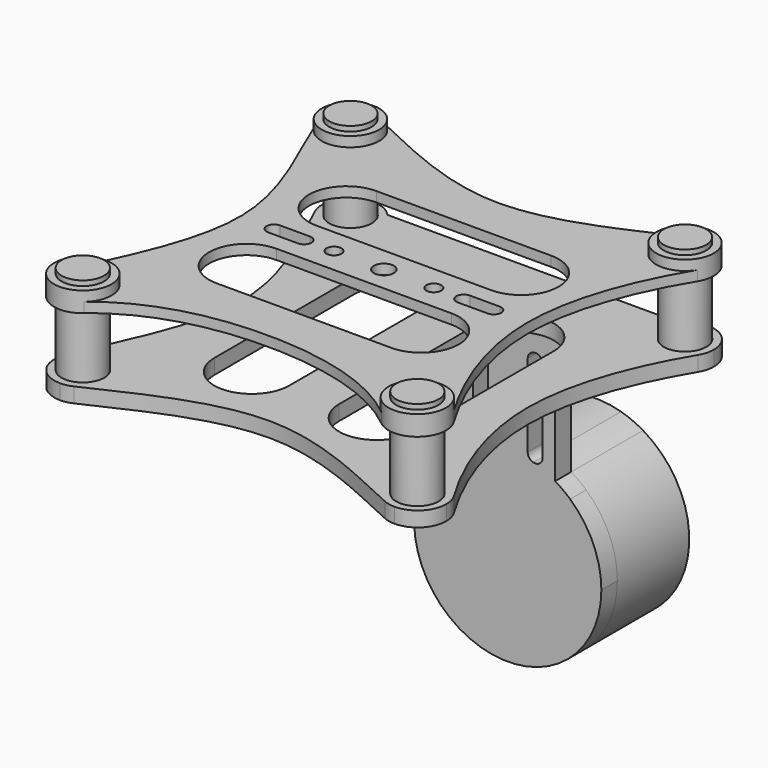
from build123d import *
from build123d import SkipClean  # not in build123d's __all__

# Parameters (mm, degrees)
F0_R          = 4.25
F0_R_2        = 1.5
F0_R_3        = 2
F1_DEPTH      = 2
F2_DEPTH      = 16
F2_DEPTH_BACK = 1
F3_R          = 4.25
F4_DEPTH      = 3
F6_START      = -31
F6_DEPTH      = 4
F8_DEPTH      = 18
F2_FACE1_R    = 4.25
F9_DEPTH      = 4


# Not quite as in the source:
# - after a boolean that leaves OpenCascade's solid faulty, fix() repairs it


with BuildPart() as f1:
    # F0 (on Top) → F1 (new body)
    with BuildSketch(Plane.XY):
        with BuildLine():
            ThreePointArc((33.5, -39.25), (37.5658639918, -37.5658639918), (39.25, -33.5))
            ThreePointArc((39.25, -33.5), (39.0420799623, -31.9677305421), (38.433356629, -30.5462748316))
            ThreePointArc((38.433356629, -30.5462748316), (29.7463089973, -29.1442791807), (29.8501801445, -37.9431199649))
            ThreePointArc((29.8501801445, -37.9431199649), (31.5616295243, -38.9134295875), (33.5, -39.25))
        make_face()
        with Locations((33.5, -33.5)):
            Circle(F0_R, mode=Mode.SUBTRACT)
        with BuildLine():
            ThreePointArc((-38.7378752338, -31.1278357908), (-39.1205107683, -32.2865921119), (-39.25, -33.5))
            ThreePointArc((-39.25, -33.5), (-37.5658639918, -37.5658639918), (-33.5, -39.25))
            ThreePointArc((-33.5, -39.25), (-31.5124151451, -38.8955543223), (-29.7698705896, -37.875915285))
            ThreePointArc((-29.7698705896, -37.875915285), (-28.2793322214, -35.9097983204), (-27.75, -33.5))
            ThreePointArc((-27.75, -33.5), (-32.2865921119, -27.8794892317), (-38.7378752338, -31.1278357908))
        make_face()
        with Locations((-33.5, -33.5)):
            Circle(F0_R, mode=Mode.SUBTRACT)
        with BuildLine():
            ThreePointArc((-31.0866116343, 38.7190091585), (-32.2644439837, 39.1156835141), (-33.5, 39.25))
            ThreePointArc((-33.5, 39.25), (-37.5658639918, 37.5658639918), (-39.25, 33.5))
            ThreePointArc((-39.25, 33.5), (-39.1467228333, 32.4150939007), (-38.8406013064, 31.369160333))
            ThreePointArc((-38.8406013064, 31.369160333), (-32.4150939007, 27.8532771667), (-27.75, 33.5))
            ThreePointArc((-27.75, 33.5), (-28.6554420685, 36.5972178562), (-31.0866116343, 38.7190091585))
        make_face()
        with Locations((-33.5, 33.5)):
            Circle(F0_R, mode=Mode.SUBTRACT)
        with BuildLine():
            ThreePointArc((39.25, 33.5), (37.5658640078, 37.5658639758), (33.5000000452, 39.25))
            ThreePointArc((33.5000000452, 39.25), (32.2902242262, 39.1212936747), (31.1346069482, 38.7409365299))
            ThreePointArc((31.1346069482, 38.7409365299), (29.1920400331, 29.691590762), (38.4113045613, 30.5097512635))
            ThreePointArc((38.4113045613, 30.5097512635), (39.036357161, 31.9471801823), (39.25, 33.5))
        make_face()
        with Locations((33.5, 33.5)):
            Circle(F0_R, mode=Mode.SUBTRACT)
        with BuildLine():
            add(Edge.make_bspline(
                [(-31.0866116343, 38.7190091585), (-21.9233343751, 34.4817016434), (0.0510624571, 22.9824943099), (21.856316187, 34.5533634934), (31.1346069482, 38.7409365299)],
                knots=[0, 0, 0, 0, 0.4997995262, 1, 1, 1, 1], degree=3))
            ThreePointArc((-31.0866116343, 38.7190091585), (-28.6554420685, 36.5972178562), (-27.75, 33.5))
            ThreePointArc((-27.75, 33.5), (-32.4150939007, 27.8532771667), (-38.8406013064, 31.369160333))
            add(Edge.make_bspline(
                [(-38.8406013064, 31.369160333), (-34.9917894272, 21.7227425064), (-22.6928169541, 0.247719594), (-34.6239443492, -22.0440393951), (-38.7378752338, -31.1278357908)],
                knots=[0, 0, 0, 0, 0.5009946988, 1, 1, 1, 1], degree=3))
            ThreePointArc((-38.7378752338, -31.1278357908), (-32.2865921119, -27.8794892317), (-27.75, -33.5))
            ThreePointArc((-27.75, -33.5), (-28.2793322214, -35.9097983204), (-29.7698705896, -37.875915285))
            add(Edge.make_bspline(
                [(29.8501801445, -37.9431199649), (21.8863357539, -31.4011860058), (0.0422874005, -26.2145083098), (-21.9031552857, -31.1701487866), (-29.7698705896, -37.875915285)],
                knots=[0, 0, 0, 0, 0.5003868235, 1, 1, 1, 1], degree=3))
            ThreePointArc((29.8501801445, -37.9431199649), (29.7463089973, -29.1442791807), (38.433356629, -30.5462748316))
            add(Edge.make_bspline(
                [(38.4113045613, 30.5097512635), (33.0474112334, 21.6998775411), (24.4241630508, -0.0411746491), (33.1042976915, -21.6455996716), (38.433356629, -30.5462748316)],
                knots=[0, 0, 0, 0, 0.4998380949, 1, 1, 1, 1], degree=3))
            ThreePointArc((38.4113045613, 30.5097512635), (29.1920400331, 29.691590762), (31.1346069482, 38.7409365299))
        make_face()
        with BuildLine():
            ThreePointArc((-17.5, -20), (-25, -12.5), (-17.5, -5))
            Line((-17.5, -5), (17.5, -5))
            ThreePointArc((17.5, -5), (22.8033008589, -7.1966991411), (25, -12.5))
            ThreePointArc((25, -12.5), (22.8033008589, -17.8033008589), (17.5, -20))
            Line((17.5, -20), (-17.5, -20))
        make_face(mode=Mode.SUBTRACT)
        with BuildLine():
            ThreePointArc((-16, 1.5), (-14.9393398282, 1.0606601718), (-14.5, 0))
            ThreePointArc((-14.5, 0), (-14.9393398282, -1.0606601718), (-16, -1.5))
            Line((-16, -1.5), (-22, -1.5))
            ThreePointArc((-22, -1.5), (-23.5, 0), (-22, 1.5))
            Line((-22, 1.5), (-16, 1.5))
        make_face(mode=Mode.SUBTRACT)
        with Locations((-10, 0)):
            Circle(F0_R_2, mode=Mode.SUBTRACT)
        Circle(F0_R_3, mode=Mode.SUBTRACT)
        with Locations((10, 0)):
            Circle(F0_R_2, mode=Mode.SUBTRACT)
        with BuildLine():
            ThreePointArc((16, -1.5), (14.5, 0), (16, 1.5))
            Line((16, 1.5), (22, 1.5))
            ThreePointArc((22, 1.5), (23.0606601718, 1.0606601718), (23.5, 0))
            ThreePointArc((23.5, 0), (23.0606601718, -1.0606601718), (22, -1.5))
            Line((22, -1.5), (16, -1.5))
        make_face(mode=Mode.SUBTRACT)
        with BuildLine():
            ThreePointArc((17.5, 20), (22.8033008589, 17.8033008589), (25, 12.5))
            ThreePointArc((25, 12.5), (22.8033008589, 7.1966991411), (17.5, 5))
            Line((17.5, 5), (-17.5, 5))
            ThreePointArc((-17.5, 5), (-25, 12.5), (-17.5, 20))
            Line((-17.5, 20), (17.5, 20))
        make_face(mode=Mode.SUBTRACT)
    extrude(amount=F1_DEPTH)

    # F0 (on Top) → F2 (join, two sides)
    with BuildSketch(Plane.XY) as f2_sk:
        with Locations((-33.5, 33.5)):
            Circle(F0_R)
        with Locations((33.5, 33.5)):
            Circle(F0_R)
        with Locations((33.5, -33.5)):
            Circle(F0_R)
        with Locations((-33.5, -33.5)):
            Circle(F0_R)
    extrude(amount=-F2_DEPTH)
    extrude(f2_sk.sketch, amount=F2_DEPTH_BACK)

    # F3 (on face) → F4 (join)
    with BuildSketch(Plane(origin=(0, 0, -16), x_dir=(1, 0, 0), z_dir=(0, 0, -1))):
        with BuildLine():
            ThreePointArc((-31.0730560074, 38.6877375668), (-32.2508883568, 39.0844119224), (-33.4864443731, 39.2187284083))
            ThreePointArc((-33.4864443731, 39.2187284083), (-37.5523083649, 37.5345924001), (-39.2364443731, 33.4687284083))
            ThreePointArc((-39.2364443731, 33.4687284083), (-39.1331672063, 32.383822309), (-38.8270456794, 31.3378887413))
            ThreePointArc((-38.8270456794, 31.3378887413), (-32.4015382738, 27.822005575), (-27.7364443731, 33.4687284083))
            ThreePointArc((-27.7364443731, 33.4687284083), (-28.6418864416, 36.5659462645), (-31.0730560074, 38.6877375668))
        make_face()
        with BuildLine():
            ThreePointArc((-29.5938515968, 35.1746655343), (-29.3267557249, 34.3402158439), (-29.2364443731, 33.4687284083))
            ThreePointArc((-29.2364443731, 33.4687284083), (-32.6316434354, 29.3055787164), (-37.3925927763, 31.794062874))
            ThreePointArc((-37.3925927763, 31.794062874), (-35.190314919, 37.3994019381), (-29.5938515968, 35.1746655343))
        make_face(mode=Mode.SUBTRACT)
        with BuildLine():
            ThreePointArc((39.2635556269, 33.4687284083), (37.5794196491, 37.5345923698), (33.5135557127, 39.2187284083))
            ThreePointArc((33.5135557127, 39.2187284083), (32.3037798729, 39.0900220873), (31.1481625752, 38.7096649382))
            ThreePointArc((31.1481625752, 38.7096649382), (29.2055956601, 29.6603191704), (38.4248601882, 30.4784796718))
            ThreePointArc((38.4248601882, 30.4784796718), (39.0499127879, 31.9159085906), (39.2635556269, 33.4687284083))
        make_face()
        with Locations((33.5135556269, 33.4687284083)):
            Circle(F3_R, mode=Mode.SUBTRACT)
        with BuildLine():
            add(Edge.make_bspline(
                [(-31.0730560074, 38.6877375668), (-21.9097787481, 34.4504300517), (0.0646180841, 22.9512227182), (21.869871814, 34.5220919017), (31.1481625752, 38.7096649382)],
                knots=[0, 0, 0, 0, 0.4997995262, 1, 1, 1, 1], degree=3))
            ThreePointArc((-31.0730560074, 38.6877375668), (-28.6418864416, 36.5659462645), (-27.7364443731, 33.4687284083))
            ThreePointArc((-27.7364443731, 33.4687284083), (-32.4015382738, 27.822005575), (-38.8270456794, 31.3378887413))
            add(Edge.make_bspline(
                [(-38.8270456794, 31.3378887413), (-34.9782338003, 21.6914709147), (-22.6792613272, 0.2164480023), (-34.6103887223, -22.0753109868), (-38.7243196068, -31.1591073825)],
                knots=[0, 0, 0, 0, 0.5009946988, 1, 1, 1, 1], degree=3))
            ThreePointArc((-38.7243196068, -31.1591073825), (-32.2730364849, -27.9107608233), (-27.7364443731, -33.5312715917))
            ThreePointArc((-27.7364443731, -33.5312715917), (-28.0954255025, -35.5311254707), (-29.1275454295, -37.2812715917))
            Line((-29.1275454295, -37.2812715917), (29.1546566834, -37.2812715917))
            ThreePointArc((29.1546566834, -37.2812715917), (30.1494089013, -28.86811635), (38.446912256, -30.5775464233))
            add(Edge.make_bspline(
                [(38.4248601882, 30.4784796718), (33.0609668604, 21.6686059494), (24.4377186777, -0.0724462408), (33.1178533184, -21.6768712633), (38.446912256, -30.5775464233)],
                knots=[0, 0, 0, 0, 0.4998380949, 1, 1, 1, 1], degree=3))
            ThreePointArc((38.4248601882, 30.4784796718), (29.2055956601, 29.6603191704), (31.1481625752, 38.7096649382))
        make_face()
        with BuildLine():
            ThreePointArc((5.0135556269, 17.4687284083), (12.5135556269, 24.9687284083), (20.0135556269, 17.4687284083))
            Line((20.0135556269, 17.4687284083), (20.0135556269, -17.5312715917))
            ThreePointArc((20.0135556269, -17.5312715917), (12.5135556269, -25.0312715917), (5.0135556269, -17.5312715917))
            Line((5.0135556269, -17.5312715917), (5.0135556269, 17.4687284083))
        make_face(mode=Mode.SUBTRACT)
        with BuildLine():
            ThreePointArc((-19.9864443731, 17.4687284083), (-12.4864443731, 24.9687284083), (-4.9864443731, 17.4687284083))
            Line((-4.9864443731, 17.4687284083), (-4.9864443731, -17.5312715917))
            ThreePointArc((-4.9864443731, -17.5312715917), (-12.4864443731, -25.0312715917), (-19.9864443731, -17.5312715917))
            Line((-19.9864443731, -17.5312715917), (-19.9864443731, 17.4687284083))
        make_face(mode=Mode.SUBTRACT)
        with BuildLine():
            ThreePointArc((-38.7243196068, -31.1591073825), (-39.1069551414, -32.3178637036), (-39.2364443731, -33.5312715917))
            ThreePointArc((-39.2364443731, -33.5312715917), (-37.5523083649, -37.5971355835), (-33.4864443731, -39.2812715917))
            ThreePointArc((-33.4864443731, -39.2812715917), (-31.0885286114, -38.7574078318), (-29.1275454295, -37.2812715917))
            ThreePointArc((-29.1275454295, -37.2812715917), (-28.0954255025, -35.5311254707), (-27.7364443731, -33.5312715917))
            ThreePointArc((-27.7364443731, -33.5312715917), (-32.2730364849, -27.9107608233), (-38.7243196068, -31.1591073825))
        make_face()
        with Locations((-33.4864443731, -33.5312715917)):
            Circle(F3_R, mode=Mode.SUBTRACT)
        with BuildLine():
            ThreePointArc((33.5135556269, -39.2812715917), (37.5794196188, -37.5971355835), (39.2635556269, -33.5312715917))
            ThreePointArc((39.2635556269, -33.5312715917), (39.0556355892, -31.9990021338), (38.446912256, -30.5775464233))
            ThreePointArc((38.446912256, -30.5775464233), (30.1494089013, -28.86811635), (29.1546566834, -37.2812715917))
            ThreePointArc((29.1546566834, -37.2812715917), (31.1156398653, -38.7574078318), (33.5135556269, -39.2812715917))
        make_face()
        with Locations((33.5135556269, -33.5312715917)):
            Circle(F3_R, mode=Mode.SUBTRACT)
        with BuildLine():
            ThreePointArc((-37.3925927763, 31.794062874), (-35.1767592921, 37.3681303464), (-29.5938515968, 35.1746655343))
            ThreePointArc((-29.5938515968, 35.1746655343), (-35.190314919, 37.3994019381), (-37.3925927763, 31.794062874))
        make_face()
    extrude(amount=-F4_DEPTH)

    # F5 (on Front) → F6 (join)
    with BuildSketch(Plane.XZ.offset(F6_START)):
        with BuildLine():
            Line((9.5, -25), (12.5, -22))
            Line((12.5, -22), (12.5, -16))
            Line((12.5, -16), (-12.5, -16))
            Line((-12.5, -16), (-12.5, -22))
            Line((-12.5, -22), (-9.5, -25))
            Line((-9.5, -25), (-7, -25))
            ThreePointArc((-7, -25), (-5.5, -23.5), (-4, -25))
            Line((-4, -25), (4, -25))
            ThreePointArc((4, -25), (5.5, -23.5), (7, -25))
            Line((7, -25), (9.5, -25))
        make_face()
        with BuildLine():
            ThreePointArc((-5.0925924775, -42.954834391), (1.99e-08, -42.25), (5.0925925158, -42.9548344018))
            ThreePointArc((5.0925925158, -42.9548344018), (4.3039416347, -42.4164528531), (4, -41.5112211773))
            Line((4, -41.5112211773), (4, -25))
            Line((4, -25), (-4, -25))
            Line((-4, -25), (-4, -41.5112211773))
            ThreePointArc((-4, -41.5112211773), (-4.3039416227, -42.4164528372), (-5.0925924775, -42.954834391))
        make_face()
        with BuildLine():
            Line((-9.5, -25), (-9.5, -44.8348368397))
            ThreePointArc((-9.5, -44.8348368397), (-7.3565984739, -43.7534653077), (-5.0925924775, -42.954834391))
            ThreePointArc((-5.0925924775, -42.954834391), (-6.4052316599, -42.7072795546), (-7, -41.5112211773))
            Line((-7, -41.5112211773), (-7, -25))
            Line((-7, -25), (-9.5, -25))
        make_face()
        with BuildLine():
            ThreePointArc((5.0925925158, -42.9548344018), (7.3565984922, -43.7534653155), (9.5, -44.8348368397))
            Line((9.5, -44.8348368397), (9.5, -25))
            Line((9.5, -25), (7, -25))
            Line((7, -25), (7, -41.5112211773))
            ThreePointArc((7, -41.5112211773), (6.4052316758, -42.7072795426), (5.0925925158, -42.9548344018))
        make_face()
        with BuildLine():
            Line((9.5, -55), (9.5, -44.8348368397))
            ThreePointArc((9.5, -44.8348368397), (7.3565984922, -43.7534653155), (5.0925925158, -42.9548344018))
            ThreePointArc((5.0925925158, -42.9548344018), (1.99e-08, -42.25), (-5.0925924775, -42.954834391))
            ThreePointArc((-5.0925924775, -42.954834391), (-7.3565984739, -43.7534653077), (-9.5, -44.8348368397))
            Line((-9.5, -44.8348368397), (-9.5, -55))
            Line((-9.5, -55), (9.5, -55))
        make_face()
        with BuildLine():
            Line((12.5, -61), (12.5, -47.0245751406))
            ThreePointArc((12.5, -47.0245751406), (11.0543538236, -45.8552397991), (9.5, -44.8348368397))
            Line((9.5, -44.8348368397), (9.5, -55))
            Line((9.5, -55), (-9.5, -55))
            Line((-9.5, -55), (-9.5, -44.8348368397))
            ThreePointArc((-9.5, -44.8348368397), (-11.0543538236, -45.8552397991), (-12.5, -47.0245751406))
            Line((-12.5, -47.0245751406), (-12.5, -61))
            Line((-12.5, -61), (12.5, -61))
        make_face()
        with BuildLine():
            ThreePointArc((-12.5, -47.0245751406), (-7.6546554462, -78.116329922), (18.75, -61))
            ThreePointArc((18.75, -61), (17.116329922, -53.3453445538), (12.5, -47.0245751406))
            Line((12.5, -47.0245751406), (12.5, -61))
            Line((12.5, -61), (-12.5, -61))
            Line((-12.5, -61), (-12.5, -47.0245751406))
        make_face()
    extrude(amount=-F6_DEPTH)

    # F7 (on face) → F8 (join)
    with BuildSketch(Plane(origin=(0, 35, 0), x_dir=(-1, 0, 0), z_dir=(0, 1, 0))):
        with BuildLine():
            ThreePointArc((-9.5, -44.8348368397), (-9.3122902661, -77.2740207079), (18.75, -61))
            ThreePointArc((18.75, -61), (16.2740207079, -51.6877097339), (9.5, -44.8348368397))
            ThreePointArc((9.5, -44.8348368397), (7.356598521, -43.7534653278), (5.0925925763, -42.9548344188))
            ThreePointArc((5.0925925763, -42.9548344188), (-8.49e-08, -42.25), (-5.0925927397, -42.9548344649))
            ThreePointArc((-5.0925927397, -42.9548344649), (-7.3565985992, -43.7534653611), (-9.5, -44.8348368397))
        make_face()
    with SkipClean():  # cleaning this boolean's faces spoils the solid; the shape is the same uncleaned
        extrude(amount=F8_DEPTH)

    # F0 (on Top) + F2_face1 (on face) → F9 (join)
    with BuildSketch(Plane.XY):
        with BuildLine():
            ThreePointArc((-38.7378752338, -31.1278357908), (-39.1205107683, -32.2865921119), (-39.25, -33.5))
            ThreePointArc((-39.25, -33.5), (-37.5658639918, -37.5658639918), (-33.5, -39.25))
            ThreePointArc((-33.5, -39.25), (-31.5124151451, -38.8955543223), (-29.7698705896, -37.875915285))
            ThreePointArc((-29.7698705896, -37.875915285), (-28.2793322214, -35.9097983204), (-27.75, -33.5))
            ThreePointArc((-27.75, -33.5), (-32.2865921119, -27.8794892317), (-38.7378752338, -31.1278357908))
        make_face()
        with Locations((-33.5, -33.5)):
            Circle(F0_R, mode=Mode.SUBTRACT)
        with BuildLine():
            ThreePointArc((33.5, -39.25), (37.5658639918, -37.5658639918), (39.25, -33.5))
            ThreePointArc((39.25, -33.5), (39.0420799623, -31.9677305421), (38.433356629, -30.5462748316))
            ThreePointArc((38.433356629, -30.5462748316), (29.7463089973, -29.1442791807), (29.8501801445, -37.9431199649))
            ThreePointArc((29.8501801445, -37.9431199649), (31.5616295243, -38.9134295875), (33.5, -39.25))
        make_face()
        with Locations((33.5, -33.5)):
            Circle(F0_R, mode=Mode.SUBTRACT)
        with BuildLine():
            ThreePointArc((-31.0866116343, 38.7190091585), (-32.2644439837, 39.1156835141), (-33.5, 39.25))
            ThreePointArc((-33.5, 39.25), (-37.5658639918, 37.5658639918), (-39.25, 33.5))
            ThreePointArc((-39.25, 33.5), (-39.1467228333, 32.4150939007), (-38.8406013064, 31.369160333))
            ThreePointArc((-38.8406013064, 31.369160333), (-32.4150939007, 27.8532771667), (-27.75, 33.5))
            ThreePointArc((-27.75, 33.5), (-28.6554420685, 36.5972178562), (-31.0866116343, 38.7190091585))
        make_face()
        with Locations((-33.5, 33.5)):
            Circle(F0_R, mode=Mode.SUBTRACT)
        with BuildLine():
            ThreePointArc((39.25, 33.5), (37.5658640078, 37.5658639758), (33.5000000452, 39.25))
            ThreePointArc((33.5000000452, 39.25), (32.2902242262, 39.1212936747), (31.1346069482, 38.7409365299))
            ThreePointArc((31.1346069482, 38.7409365299), (29.1920400331, 29.691590762), (38.4113045613, 30.5097512635))
            ThreePointArc((38.4113045613, 30.5097512635), (39.036357161, 31.9471801823), (39.25, 33.5))
        make_face()
        with Locations((33.5, 33.5)):
            Circle(F0_R, mode=Mode.SUBTRACT)
    with BuildSketch(Plane(origin=(-33.5, -33.5, 1), x_dir=(1, 0, 0), z_dir=(0, 0, 1))):
        Circle(F2_FACE1_R)
        with Locations((0, 67)):
            Circle(F2_FACE1_R)
        with Locations((67, 67)):
            Circle(F2_FACE1_R)
        with Locations((67, 0)):
            Circle(F2_FACE1_R)
    extrude(amount=F9_DEPTH)

    add(f1.part.fix(), mode=Mode.REPLACE)


solid = f1.part
